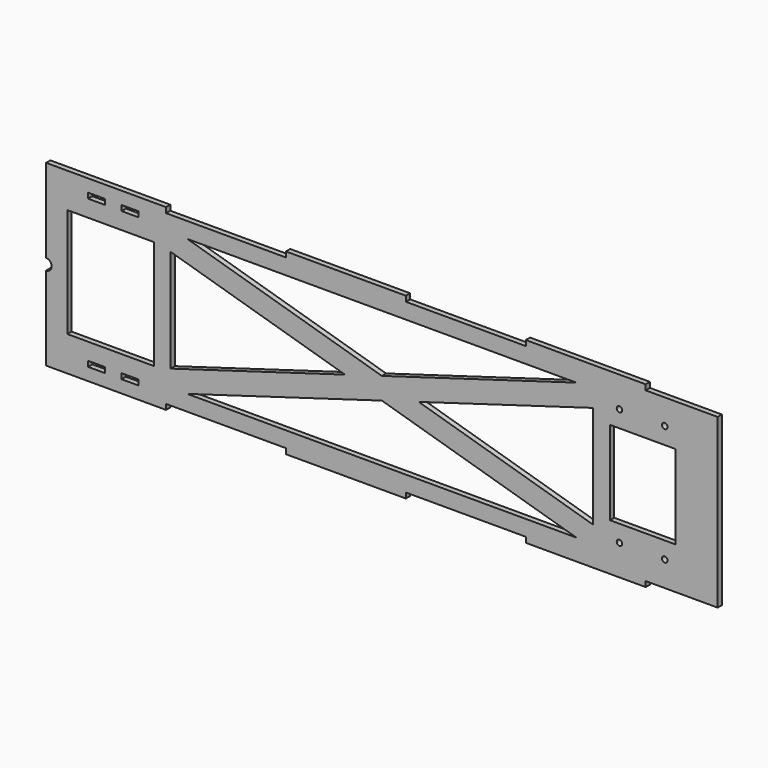
from build123d import *

# Parameters (mm, degrees)
F0_W     = 10
F0_H     = 3.175
F0_W_2   = 51.432349664
F0_H_2   = 65
F0_R     = 1.64084
F0_W_3   = 39.0626990616
F0_H_3   = 50
F1_DEPTH = 3.175


# Not quite as in the source:
# - a feature names something its author has since deleted; it is built from what else it names


with BuildPart() as f1:
    # F0 (on Front) → F1 (new body)
    with BuildSketch(Plane.XZ):
        with BuildLine():
            Line((79.2994276966, -35.2024036679), (122.1565705538, -35.2024036679))
            Line((122.1565705538, -35.2024036679), (122.1565705538, 64.7975963321))
            Line((122.1565705538, 64.7975963321), (79.2994276966, 64.7975963321))
            Line((79.2994276966, 64.7975963321), (79.2994276966, 67.9725963321))
            Line((79.2994276966, 67.9725963321), (7.870856268, 67.9725963321))
            Line((7.870856268, 67.9725963321), (7.870856268, 64.7975963321))
            Line((7.870856268, 64.7975963321), (-63.5577151605, 64.7975963321))
            Line((-63.5577151605, 64.7975963321), (-63.5577151605, 67.9725963321))
            Line((-63.5577151605, 67.9725963321), (-134.9862865891, 67.9725963321))
            Line((-134.9862865891, 67.9725963321), (-134.9862865891, 64.7975963321))
            Line((-134.9862865891, 64.7975963321), (-206.4148580177, 64.7975963321))
            Line((-206.4148580177, 64.7975963321), (-206.4148580177, 67.9725963321))
            Line((-206.4148580177, 67.9725963321), (-277.8434294462, 67.9725963321))
            Line((-277.8434294462, 67.9725963321), (-277.8434294462, 64.7975963321))
            Line((-277.8434294462, 64.7975963321), (-277.8434294462, 18.0995963321))
            ThreePointArc((-277.8434294462, 18.0995963321), (-275.5085628548, 17.1324629236), (-274.5414294462, 14.7975963321))
            ThreePointArc((-274.5414294462, 14.7975963321), (-275.5085628548, 12.4627297406), (-277.8434294462, 11.4955963321))
            Line((-277.8434294462, 11.4955963321), (-277.8434294462, -35.2024036679))
            Line((-277.8434294462, -35.2024036679), (-277.8434294462, -38.3774036679))
            Line((-277.8434294462, -38.3774036679), (-206.4148580177, -38.3774036679))
            Line((-206.4148580177, -38.3774036679), (-206.4148580177, -35.2024036679))
            Line((-206.4148580177, -35.2024036679), (-134.9862865891, -35.2024036679))
            Line((-134.9862865891, -35.2024036679), (-134.9862865891, -38.3774036679))
            Line((-134.9862865891, -38.3774036679), (-63.5577151605, -38.3774036679))
            Line((-63.5577151605, -38.3774036679), (-63.5577151605, -35.2024036679))
            Line((-63.5577151605, -35.2024036679), (7.870856268, -35.2024036679))
            Line((7.870856268, -35.2024036679), (7.870856268, -38.3774036679))
            Line((7.870856268, -38.3774036679), (79.2994276966, -38.3774036679))
            Line((79.2994276966, -38.3774036679), (79.2994276966, -35.2024036679))
        make_face()
        with Locations((-247.8332173824, -29.2899036679)):
            Rectangle(F0_W, F0_H, mode=Mode.SUBTRACT)
        with Locations((-227.8332173824, -29.2899036679)):
            Rectangle(F0_W, F0_H, mode=Mode.SUBTRACT)
        with Locations((-239.4272546143, 14.7975963321)):
            Rectangle(F0_W_2, F0_H_2, mode=Mode.SUBTRACT)
        with Locations((63.6818705538, -20.2024036679)):
            Circle(F0_R, mode=Mode.SUBTRACT)
        with Locations((90.6312705538, -20.2024036679)):
            Circle(F0_R, mode=Mode.SUBTRACT)
        Polygon((48.0242208898, -15.8320336679), (48.0242208898, -25.8320336679), (38.0242208898, -25.8320336679), (-193.7110797823, -25.8320336679), (-203.7110797823, -25.8320336679), (-203.7110797823, -15.8320336679), (-203.7110797823, 45.4272263321), (-203.7110797823, 55.4272263321), (-193.7110797823, 55.4272263321), (38.0242208898, 55.4272263321), (48.0242208898, 55.4272263321), (48.0242208898, 45.4272263321), align=None, mode=Mode.SUBTRACT)
        with Locations((77.5555704206, 14.7975963321)):
            Rectangle(F0_W_3, F0_H_3, mode=Mode.SUBTRACT)
        with Locations((-247.8332173824, 58.8850963321)):
            Rectangle(F0_W, F0_H, mode=Mode.SUBTRACT)
        with Locations((-227.8332173824, 58.8850963321)):
            Rectangle(F0_W, F0_H, mode=Mode.SUBTRACT)
        with Locations((63.6818705538, 49.7975963321)):
            Circle(F0_R, mode=Mode.SUBTRACT)
        with Locations((90.6312705538, 49.7975963321)):
            Circle(F0_R, mode=Mode.SUBTRACT)
        Polygon((-203.7110797823, 45.4272263321), (-99.8051057724, 14.7975963321), (-77.8434294462, 21.2715072545), (-193.7110797823, 55.4272263321), (-203.7110797823, 55.4272263321), align=None)
        Polygon((-203.7110797823, -25.8320336679), (-193.7110797823, -25.8320336679), (-77.8434294462, 8.3236854097), (-99.8051057724, 14.7975963321), (-203.7110797823, -15.8320336679), align=None)
        Polygon((38.0242208898, -25.8320336679), (48.0242208898, -25.8320336679), (48.0242208898, -15.8320336679), (-55.8817531201, 14.7975963321), (-77.8434294462, 8.3236854097), align=None)
        Polygon((-55.8817531201, 14.7975963321), (48.0242208898, 45.4272263321), (48.0242208898, 55.4272263321), (38.0242208898, 55.4272263321), (-77.8434294462, 21.2715072545), align=None)
        Polygon((-99.8051057724, 14.7975963321), (-77.8434294462, 8.3236854097), (-55.8817531201, 14.7975963321), (-77.8434294462, 21.2715072545), align=None)
    extrude(amount=F1_DEPTH)


solid = f1.part
